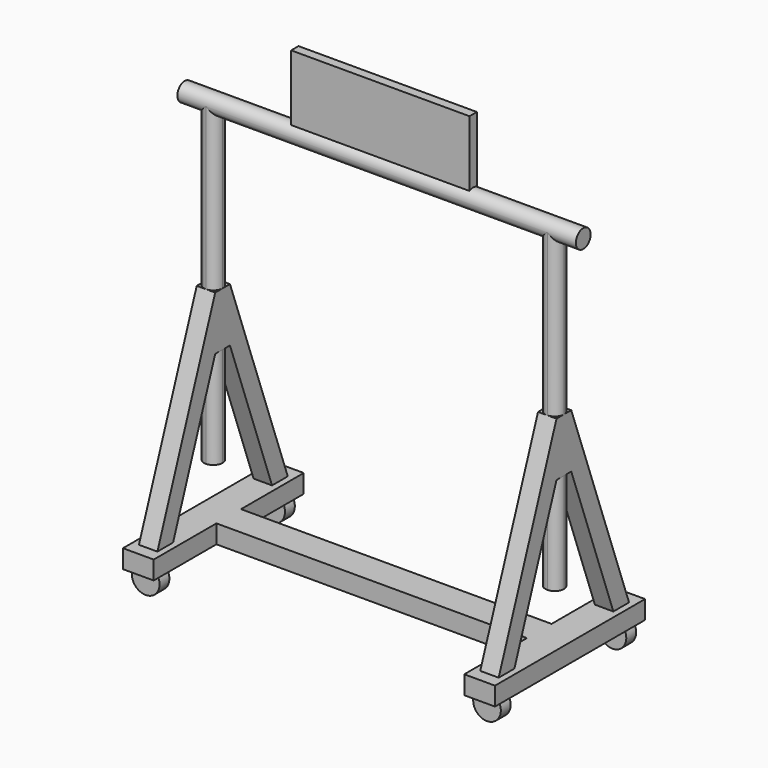
from build123d import *

# Parameters (mm, degrees)
F2_DEPTH          = 3
F6_DEPTH          = 1.5
F9_DEPTH          = 26.2
F9_DEPTH_BACK     = 25
F10_R             = 1.5
F11_DEPTH         = 32.4
F13_R             = 2.25
F14_DEPTH         = 2
F14_COPIES2_COUNT = 2
F14_COPIES2_PITCH = 61.077819
F15_W             = 29
F15_H             = 11
F16_DEPTH         = 0.75


# Not quite as in the source:
# - a pattern or mirror of a feature is missing from the dataset's text; its kind, count and spacing are read off the source's solid


with BuildPart() as f2:
    # F1 (on offset) → F2 (new body)
    with BuildSketch(Plane.XY.offset(3.5)):
        Polygon((-25.25, -15.25), (-25.25, -2.5), (-25.25, 2.5), (-25.25, 15.25), (-30.25, 15.25), (-30.25, 0), (-30.25, -15.25), align=None)
        Polygon((0, -2.5), (25.25, -2.5), (25.25, 2.5), (0, 2.5), (-25.25, 2.5), (-25.25, -2.5), align=None)
        Polygon((30.25, -15.25), (30.25, 0), (30.25, 15.25), (25.25, 15.25), (25.25, 2.5), (25.25, -2.5), (25.25, -15.25), align=None)
    extrude(amount=F2_DEPTH)

    # F5 (on plane+point) → F6 (join, symmetric)
    with BuildSketch(Plane.YZ.offset(27.75)):
        Polygon((10.057664814, 6.5), (13.25, 6.5), (1.5, 38.8), (0, 38.8), (-1.5, 38.8), (-13.25, 6.5), (-10.057664814, 6.5), (-1.5, 30.0244743399), (0, 30.0244743399), (1.5, 30.0244743399), align=None)
    f6 = extrude(amount=F6_DEPTH, both=True)

    # F6_copies: F6 across plane
    add(f6.mirror(Plane(origin=(0, 0, 0), x_dir=(0, 0, -1), z_dir=(-1, 0, 0))))

    # F8 (on face) → F9 (join, two sides)
    with BuildSketch(Plane.XY.offset(38.8)) as f9_sk:
        with BuildLine():
            ThreePointArc((27.75, -1.5), (28.8106601718, -1.0606601718), (29.25, 0))
            ThreePointArc((29.25, 0), (28.8106601718, 1.0606601718), (27.75, 1.5))
            ThreePointArc((27.75, 1.5), (26.68933982, 1.0606601636), (26.25, -2.31e-08))
            ThreePointArc((26.25, -2.31e-08), (26.6893398364, -1.06066018), (27.75, -1.5))
        make_face()
    f9 = extrude(amount=F9_DEPTH) + extrude(f9_sk.sketch, amount=-F9_DEPTH_BACK)

    # F9_copies: F9 across plane
    add(f9.mirror(Plane(origin=(0, 0, 0), x_dir=(0, 0, -1), z_dir=(-1, 0, 0))))

    # F10 (on Right) → F11 (join, symmetric)
    with BuildSketch(Plane.YZ):
        with Locations((0, 65)):
            Circle(F10_R)
    extrude(amount=F11_DEPTH, both=True)

    # F13 (on offset) → F14 (join)
    with BuildSketch(Plane.XZ.offset(13.75)):
        with Locations((27.75, 2.25)):
            Circle(F13_R)
    f14 = extrude(amount=-F14_DEPTH)

    # F14_copies: F14 across plane
    add(f14.mirror(Plane.ZX))

    # F14_copies1: F14 across plane
    add(f14.mirror(Plane(origin=(0, 0, 0), x_dir=(0, 0, -1), z_dir=(-1, 0, 0))))

    # F14_copies2: F14 ×2
    with Locations(*[Vector(-0.908676844, 0.4175001716, 0) * (i * F14_COPIES2_PITCH) for i in range(1, F14_COPIES2_COUNT)]):
        add(f14)

    # F15 (on Front) → F16 (join, symmetric)
    with BuildSketch(Plane.XZ):
        with Locations((0, 71.5)):
            Rectangle(F15_W, F15_H)
    extrude(amount=F16_DEPTH, both=True)


solid = f2.part
